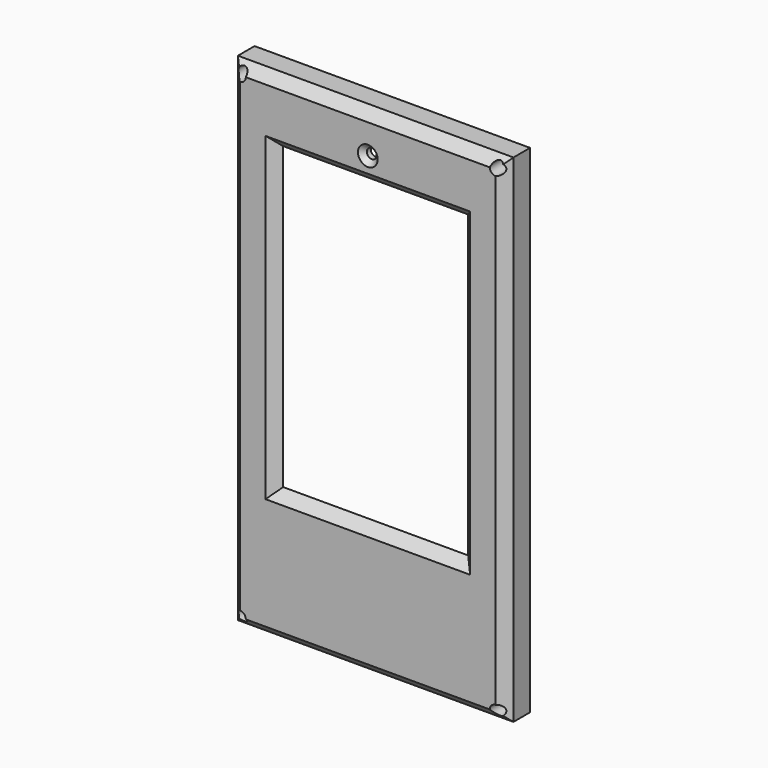
from build123d import *

# Parameters (mm, degrees)
F0_W        = 140
F0_H        = 252.5
F0_R        = 1
F0_W_2      = 94
F0_H_2      = 152.5
F0_R_2      = 2.5
F0_W_3      = 12
F0_H_3      = 34
F1_DEPTH    = 15.56
F2_DEPTH    = 10.56
F3_T1_DEPTH = 165.7168298797
F3_T3_DEPTH = 278.2168298797
F4_SIZE     = 2.5
F5_R        = 3
F6_DEPTH    = 10
F7_SIZE     = 4.99999


# Not quite as in the source:
# - a fillet or chamfer that OpenCascade refuses, or shapes differently, is made with other operations: its cross-section is extruded or revolved along the edge and cut away or added
# - a fillet or chamfer is up to 0.001 mm smaller than in the source, because OpenCascade refuses the exact size
# - a feature names something its author has since deleted; it is built from what else it names


with BuildPart() as f1:
    # F0 (on Front) → F1 (new body)
    with BuildSketch(Plane.XZ):
        with Locations((-70, 126.25)):
            Rectangle(F0_W, F0_H)
        with Locations((-135, 5)):
            Circle(F0_R, mode=Mode.SUBTRACT)
        with Locations((-5, 5)):
            Circle(F0_R, mode=Mode.SUBTRACT)
        with Locations((-135, 247.5)):
            Circle(F0_R, mode=Mode.SUBTRACT)
        Polygon((-130, 44), (-130, 242.5), (-10, 242.5), (-10, 44), (-64, 44), (-64, 10), (-76, 10), (-76, 44), align=None, mode=Mode.SUBTRACT)
        with Locations((-5, 247.5)):
            Circle(F0_R, mode=Mode.SUBTRACT)
        Polygon((-10, 242.5), (-130, 242.5), (-130, 44), (-76, 44), (-64, 44), (-10, 44), align=None)
        with Locations((-70, 143.25)):
            Rectangle(F0_W_2, F0_H_2, mode=Mode.SUBTRACT)
        with Locations((-70, 232.5)):
            Circle(F0_R_2, mode=Mode.SUBTRACT)
        with Locations((-70, 27)):
            Rectangle(F0_W_3, F0_H_3)
    extrude(amount=F1_DEPTH)

    # F0 (on Front) → F2 (cut)
    with BuildSketch(Plane.XZ):
        Polygon((-10, 242.5), (-130, 242.5), (-130, 44), (-76, 44), (-64, 44), (-10, 44), align=None)
        with Locations((-70, 143.25)):
            Rectangle(F0_W_2, F0_H_2, mode=Mode.SUBTRACT)
        with Locations((-70, 232.5)):
            Circle(F0_R_2, mode=Mode.SUBTRACT)
        with Locations((-70, 27)):
            Rectangle(F0_W_3, F0_H_3)
    extrude(amount=F2_DEPTH, mode=Mode.SUBTRACT)

    # F3: chamfer of 5 on 4 edges, made by hand

    # F3_s2 → F3_t1 (cut)
    with BuildSketch(Plane.YZ.offset(-152.8584149398)):
        Polygon((-10.56, 0), (-15.56, 5), (-15.56, 0), align=None)
        Polygon((-15.56, 247.5), (-10.56, 252.5), (-15.56, 252.5), align=None)
    extrude(amount=F3_T1_DEPTH, mode=Mode.SUBTRACT)

    # F3_s4 → F3_t3 (cut)
    with BuildSketch(Plane.XY.offset(-12.8584149398)):
        Polygon((-140, -10.56), (-135, -15.56), (-140, -15.56), align=None)
        Polygon((0, -10.56), (-5, -15.56), (0, -15.56), align=None)
    extrude(amount=F3_T3_DEPTH, mode=Mode.SUBTRACT)

    # F4
    f4_edges = [f1.edges().sort_by_distance(p)[0] for p in [
        (-72.5, -15.56, 232.5),
    ]]
    chamfer(f4_edges, length=F4_SIZE)

    # F5 (on face) → F6 (cut)
    with BuildSketch(Plane.XZ.offset(15.56)):
        with Locations((-135, 247.5)):
            Circle(F5_R)
        with Locations((-135, 5)):
            Circle(F5_R)
        with Locations((-5, 247.5)):
            Circle(F5_R)
        with Locations((-5, 5)):
            Circle(F5_R)
    extrude(amount=-F6_DEPTH, mode=Mode.SUBTRACT)

    # F7 (size 5 in the source; OpenCascade refuses exactly that, so slightly less here)
    f7_edges = [f1.edges().sort_by_distance(p)[0] for p in [
        (-70, -15.56, 67),
        (-117, -15.56, 143.25),
        (-23, -15.56, 143.25),
        (-70, -15.56, 219.5),
    ]]
    chamfer(f7_edges, length=F7_SIZE)


solid = f1.part
